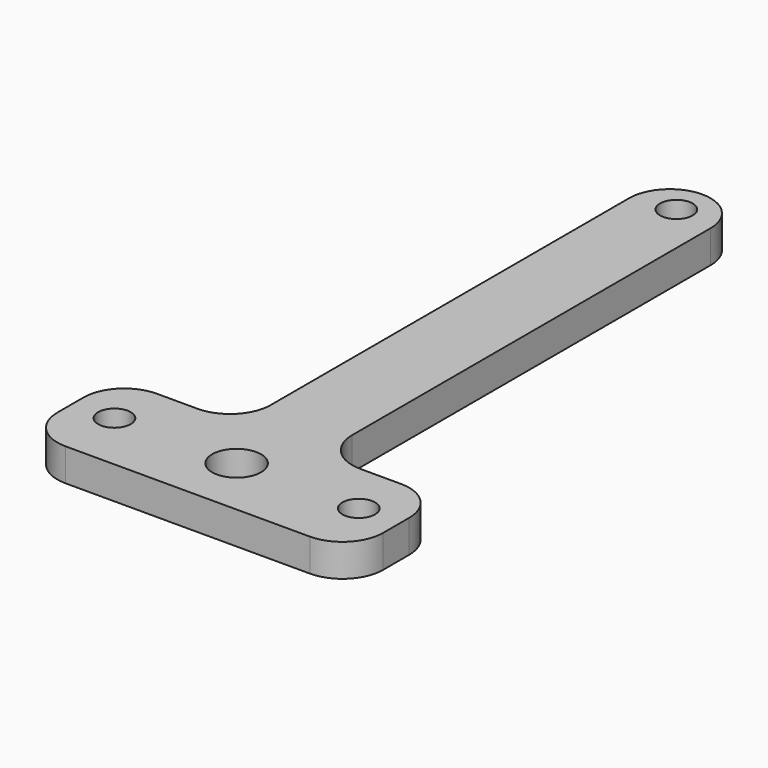
from build123d import *

# Parameters (mm, degrees)
F1_DEPTH = 4
F2_R     = 2
F2_R_2   = 3
F3_DEPTH = 25
F4_R     = 4.99999


# Not quite as in the source:
# - a fillet or chamfer is up to 0.001 mm smaller than in the source, because OpenCascade refuses the exact size


with BuildPart() as f1:
    # F0 (on Top) → F1 (new body)
    with BuildSketch(Plane.XY):
        Polygon((-20, 14), (-20, 0), (20, 0), (20, 14), (5, 14), (5, 79), (-5, 79), (-5, 14), align=None)
    extrude(amount=F1_DEPTH)

    # F2 (on Top) → F3 (cut)
    with BuildSketch(Plane.XY):
        with Locations((-15, 7.5)):
            Circle(F2_R)
        with Locations((15, 7.5)):
            Circle(F2_R)
        with Locations((0, 75)):
            Circle(F2_R)
        with Locations((0, 7.5)):
            Circle(F2_R_2)
    extrude(amount=F3_DEPTH, mode=Mode.SUBTRACT)

    # F4 (radius 5 in the source; OpenCascade refuses exactly that, so slightly less here)
    f4_edges = [f1.edges().sort_by_distance(p)[0] for p in [
        (-5, 79, 2),
        (5, 79, 2),
        (20, 0, 2),
        (-20, 0, 2),
        (-20, 14, 2),
        (20, 14, 2),
        (5, 14, 2),
        (-5, 14, 2),
    ]]
    fillet(f4_edges, radius=F4_R)


solid = f1.part
